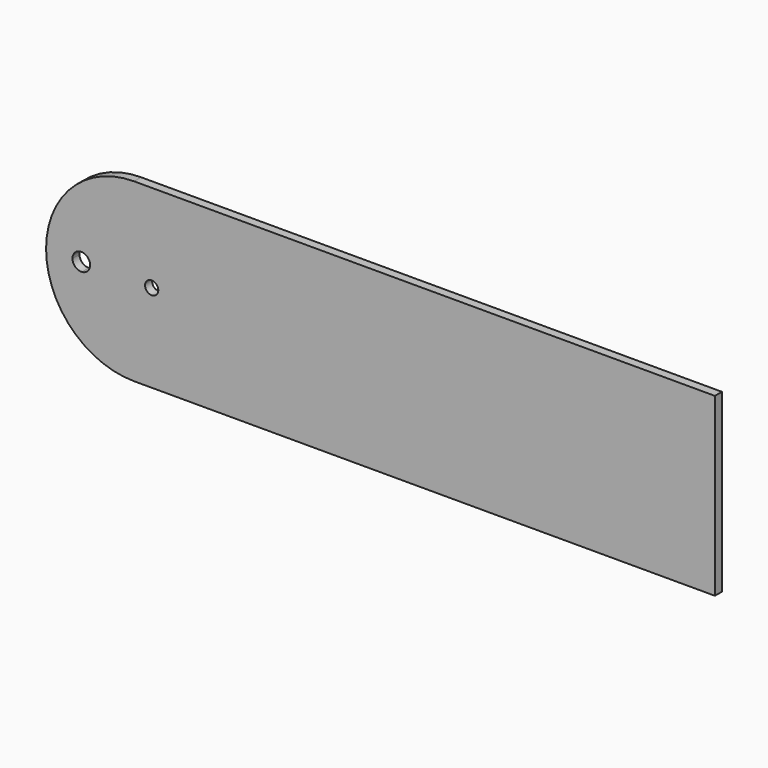
from build123d import *

# Parameters (mm, degrees)
F1_DEPTH = 3.175


# Not quite as in the source:
# - a feature names something its author has since deleted; it is built from what else it names


with BuildPart() as f1:
    # F0 (on Front) → F1 (new body)
    with BuildSketch(Plane.XZ):
        with BuildLine():
            ThreePointArc((0, 31.75), (9.2993596973, 9.2993596973), (31.75, 0))
            Line((31.75, 0), (241.3, 0))
            Line((241.3, 0), (241.3, 63.5))
            Line((241.3, 63.5), (31.75, 63.5))
            ThreePointArc((31.75, 63.5), (9.2993596973, 54.2006403027), (0, 31.75))
        make_face()
        with BuildLine():
            ThreePointArc((12.8984375, 28.5812072396), (10.5262260999, 29.4358409667), (9.525, 31.75))
            ThreePointArc((9.525, 31.75), (10.5262260999, 34.0641590333), (12.8984375, 34.9187927604))
            ThreePointArc((12.8984375, 34.9187927604), (39.6875, 57.1003420835), (63.5, 31.75))
            ThreePointArc((63.5, 31.75), (39.6875, 6.3996579165), (12.8984375, 28.5812072396))
        make_face(mode=Mode.SUBTRACT)
        with BuildLine():
            ThreePointArc((63.5, 31.75), (39.6875, 57.1003420835), (12.8984375, 34.9187927604))
            ThreePointArc((12.8984375, 34.9187927604), (15.0141590333, 33.9237739001), (15.875, 31.75))
            ThreePointArc((15.875, 31.75), (15.0141590333, 29.5762260999), (12.8984375, 28.5812072396))
            ThreePointArc((12.8984375, 28.5812072396), (39.6875, 6.3996579165), (63.5, 31.75))
        make_face()
        with BuildLine():
            ThreePointArc((40.48125, 31.75), (38.1, 29.36875), (35.71875, 31.75))
            ThreePointArc((35.71875, 31.75), (38.1, 34.13125), (40.48125, 31.75))
        make_face(mode=Mode.SUBTRACT)
    extrude(amount=F1_DEPTH)


solid = f1.part
